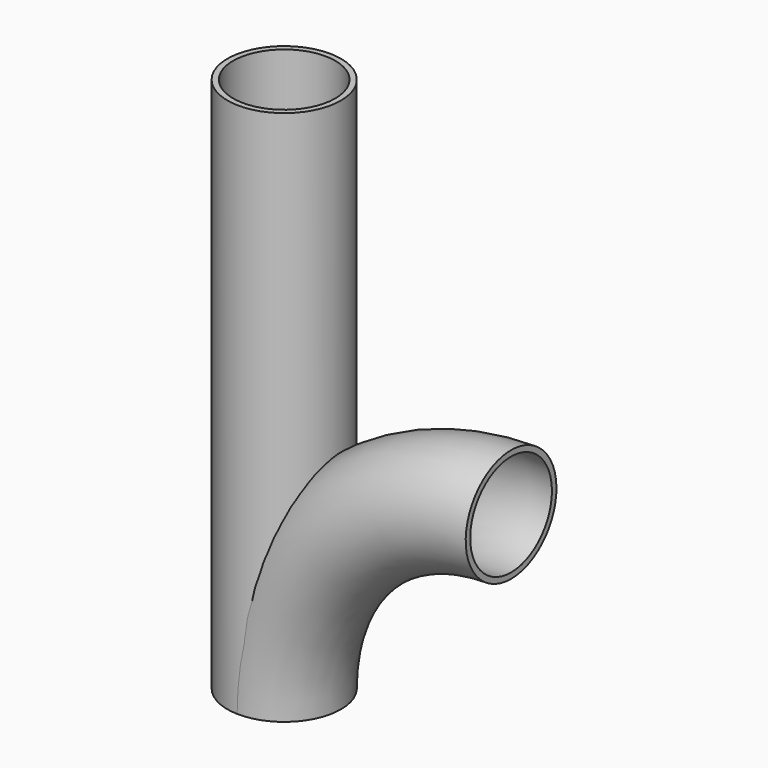
from build123d import *

# Parameters (mm, degrees)
F0_R     = 20
F1_DEPTH = 189
F3_ANGLE = 90
F4_T     = -2
F4_2_T   = -2


with BuildPart() as f1:
    # F0 (on Top) → F1 (new body)
    with BuildSketch(Plane.XY):
        Circle(F0_R)
    extrude(amount=F1_DEPTH)

    # F4#2
    f4_2_openings = [f1.faces().sort_by_distance(p)[0] for p in [
        (0, 0, 0),
        (0, 0, 189),
    ]]
    offset(amount=F4_2_T, openings=f4_2_openings)


with BuildPart() as f3:
    # F0 (on Top) → F3 (revolve)
    with BuildSketch(Plane.XY):
        Circle(F0_R)
    revolve(axis=Axis((80, 46.6175764806, 0), (0, 1, 0)), revolution_arc=F3_ANGLE)

    # F4
    f4_openings = [f3.faces().sort_by_distance(p)[0] for p in [
        (80, 0, 80),
        (0, 0, 0),
    ]]
    offset(amount=F4_T, openings=f4_openings)


solid = Compound([f1.part, f3.part])
